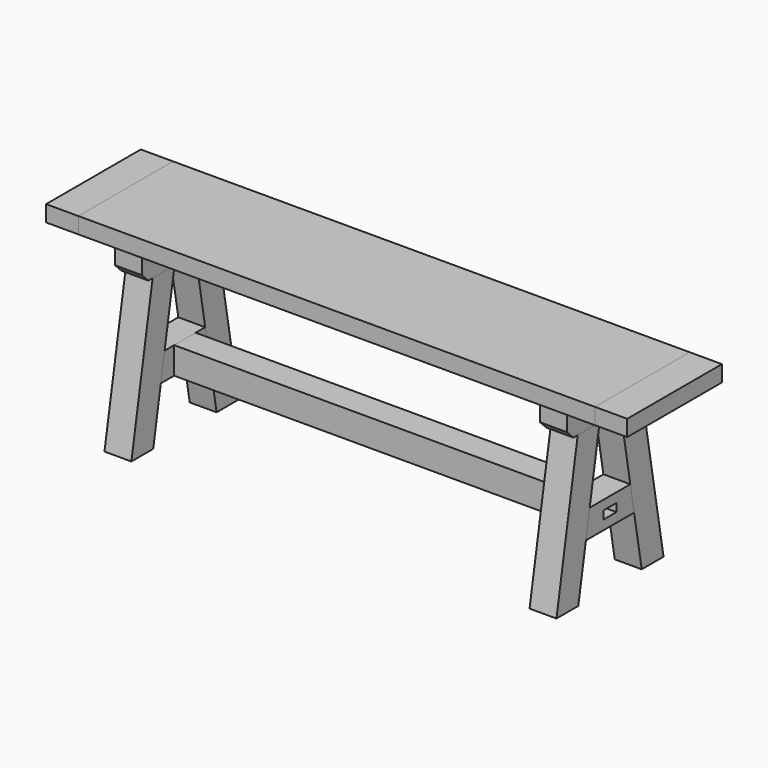
from build123d import *

# Parameters (mm, degrees)
F0_W      = 279.4
F0_H      = 38.1
F1_DEPTH  = 609.6
F2_W      = 228.6
F2_H      = 12.7
F3_DEPTH  = 38.1
F4_W      = 279.4
F4_H      = 38.1
F5_DEPTH  = 76.2
F7_START  = 6.35
F7_DEPTH  = 31.75
F9_W      = 63.5
F9_H      = 63.5
F10_DEPTH = 469.9
F11_W     = 38.1
F11_H     = 19.05
F12_DEPTH = 38.1
F15_DEPTH = 63.5
F16_DEPTH = 63.5
F17_DEPTH = 63.5
F14_W     = 63.5
F14_H     = 63.5
F14_W_2   = 38.1
F14_H_2   = 19.05
F18_DEPTH = 63.5


# Not quite as in the source:
# - a pattern or mirror of a feature is missing from the dataset's text; its kind, count and spacing are read off the source's solid


with BuildPart() as f1:
    # F0 (on Right) → F1 (new body, symmetric)
    with BuildSketch(Plane.YZ):
        with Locations((0, 438.15)):
            Rectangle(F0_W, F0_H)
    extrude(amount=F1_DEPTH, both=True)

    # F2 (on face) → F3 (join)
    with BuildSketch(Plane.YZ.offset(609.6)):
        with Locations((0, 438.15)):
            Rectangle(F2_W, F2_H)
    f3 = extrude(amount=F3_DEPTH)

    # F3_copies: F3 across plane
    add(f3.mirror(Plane(origin=(0, 0, 0), x_dir=(0, 0, -1), z_dir=(-1, 0, 0))))


with BuildPart() as f5:
    # F4 (on face) → F5 (new body)
    with BuildSketch(Plane.YZ.offset(609.6)):
        with Locations((0, 438.15)):
            Rectangle(F4_W, F4_H)
        with BuildLine():
            ThreePointArc((-120.396, 431.8), (-126.746, 438.15), (-120.396, 444.5))
            Line((-120.396, 444.5), (120.65, 444.5))
            ThreePointArc((120.65, 444.5), (127, 438.15), (120.65, 431.8))
            Line((120.65, 431.8), (-120.396, 431.8))
        make_face(mode=Mode.SUBTRACT)
    extrude(amount=F5_DEPTH)

    # F6 (on face) → F7 (join)
    with BuildSketch(Plane.YZ.offset(647.7).offset(F7_START)):
        with BuildLine():
            ThreePointArc((-120.396, 444.5), (-126.746, 438.15), (-120.396, 431.8))
            Line((-120.396, 431.8), (120.65, 431.8))
            ThreePointArc((120.65, 431.8), (127, 438.15), (120.65, 444.5))
            Line((120.65, 444.5), (-120.396, 444.5))
        make_face()
    extrude(amount=F7_DEPTH)


with BuildPart() as f8_1:
    # F8: instance of F5
    add(f5.part.mirror(Plane.YZ))


with BuildPart() as f10:
    # F9 (on Right) → F10 (new body, symmetric)
    with BuildSketch(Plane.YZ):
        with Locations((0, 158.75)):
            Rectangle(F9_W, F9_H)
    extrude(amount=F10_DEPTH, both=True)

    # F11 (on face) → F12 (join)
    with BuildSketch(Plane.YZ.offset(469.9)):
        with Locations((0, 158.75)):
            Rectangle(F11_W, F11_H)
    extrude(amount=F12_DEPTH)

    # F13: F10 across plane


with BuildPart() as f10_1:
    add(f10.part)
    add(f10.part.mirror(Plane.YZ))


with BuildPart() as f15:
    # F14 (on face) → F15 (new body)
    with BuildSketch(Plane.YZ.offset(469.9)):
        Polygon((-107.95, 355.6), (-95.25, 355.6), (-30.7704101453, 355.6), (30.7704101453, 355.6), (95.25, 355.6), (107.95, 355.6), (127, 374.65), (127, 419.1), (-127, 419.1), (-127, 374.65), align=None)
    extrude(amount=F15_DEPTH)


with BuildPart() as f16:
    # F14 (on face) → F16 (new body, through all)
    with BuildSketch(Plane.YZ.offset(469.9)):
        Polygon((-95.25, 355.6), (-157.9518743399, 0), (-93.4722844852, 0), (-71.0787579352, 127), (-59.8819946602, 190.5), (-30.7704101453, 355.6), align=None)
    extrude(amount=F16_DEPTH)


with BuildPart() as f17:
    # F14 (on face) → F17 (new body, through all)
    with BuildSketch(Plane.YZ.offset(469.9)):
        Polygon((95.25, 355.6), (30.7704101453, 355.6), (59.8819946602, 190.5), (71.0787579352, 127), (93.4722844852, 0), (157.9518743399, 0), align=None)
    extrude(amount=F17_DEPTH)


with BuildPart() as f18:
    # F14 (on face) → F18 (new body, through all)
    with BuildSketch(Plane.YZ.offset(469.9)):
        Polygon((-59.8819946602, 190.5), (-71.0787579352, 127), (-31.75, 127), (-31.75, 190.5), align=None)
        with Locations((0, 158.75)):
            Rectangle(F14_W, F14_H)
        with Locations((0, 158.75)):
            Rectangle(F14_W_2, F14_H_2, mode=Mode.SUBTRACT)
        Polygon((31.75, 190.5), (31.75, 127), (71.0787579352, 127), (59.8819946602, 190.5), align=None)
    extrude(amount=F18_DEPTH)


with BuildPart() as f19_1:
    # F19: instance of F16
    add(f16.part.mirror(Plane.YZ))


with BuildPart() as f19_2:
    # F19: instance of F15
    add(f15.part.mirror(Plane.YZ))


with BuildPart() as f19_3:
    # F19: instance of F17
    add(f17.part.mirror(Plane.YZ))


with BuildPart() as f19_4:
    # F19: instance of F18
    add(f18.part.mirror(Plane.YZ))


solid = Compound([f1.part, f5.part, f8_1.part, f10_1.part, f15.part, f16.part, f17.part, f18.part, f19_1.part, f19_2.part, f19_3.part, f19_4.part])
